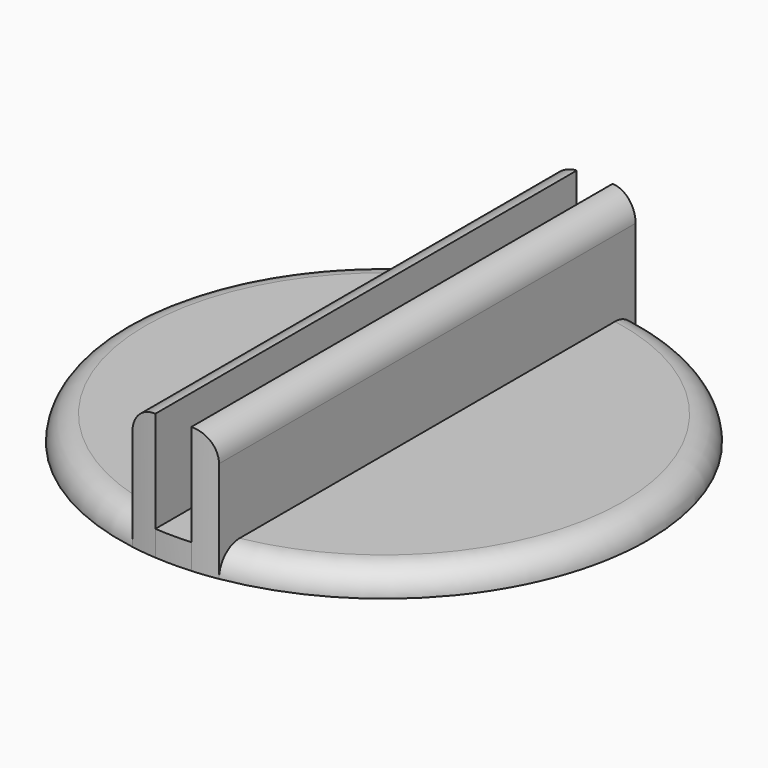
from build123d import *

# Parameters (mm, degrees)
F1_DEPTH      = 1.2
F2_DEPTH      = 6
F3_T2_ANGLE   = 188.6591090802
F3_2_T2_ANGLE = 188.6591090802
F3_3_T1_DEPTH = 30.6615084697
F3_4_T1_DEPTH = 30.6615084697


# Not quite as in the source:
# - a fillet or chamfer that OpenCascade refuses, or shapes differently, is made with other operations: its cross-section is extruded or revolved along the edge and cut away or added


with BuildPart() as f1:
    # F0 (on Top) → F1 (new body)
    with BuildSketch(Plane.XY):
        with BuildLine():
            Line((-2.05, -12.3307542348), (-2.05, 12.3307542348))
            ThreePointArc((-2.05, 12.3307542348), (-12.5, 0), (-2.05, -12.3307542348))
        make_face()
    extrude(amount=F1_DEPTH)

    # F3: fillet of radius 1.2 on 1 edges, made by hand

    # F3_s1 → F3_t2 (revolve, cut)
    with BuildSketch(Plane(origin=(0, 0, 0), x_dir=(0, 0, 1), z_dir=(0.997146325, -0.0754930889, 0))):
        with BuildLine():
            ThreePointArc((0, -12.5), (0.8485281374, -12.1485281374), (1.2, -11.3))
            Line((1.2, -11.3), (1.2, -12.5))
            Line((1.2, -12.5), (0, -12.5))
        make_face()
    revolve(axis=Axis((0, 0, 1.2), (0, 0, 1)), revolution_arc=F3_T2_ANGLE, mode=Mode.SUBTRACT)


with BuildPart() as f1b:
    # F0 (on Top) → F1, piece 2 (new body)
    with BuildSketch(Plane.XY):
        with BuildLine():
            Line((0.85, -12.4710665141), (0.85, 12.4710665141))
            ThreePointArc((0.85, 12.4710665141), (0, 12.5), (-0.85, 12.4710665141))
            Line((-0.85, 12.4710665141), (-0.85, -12.4710665141))
            ThreePointArc((-0.85, -12.4710665141), (0, -12.5), (0.85, -12.4710665141))
        make_face()
    extrude(amount=F1_DEPTH)


with BuildPart() as f1c:
    # F0 (on Top) → F1, piece 3 (new body)
    with BuildSketch(Plane.XY):
        with BuildLine():
            ThreePointArc((2.05, -12.3307542348), (9.5361155614, -8.0816149376), (12.5, 0))
            ThreePointArc((12.5, 0), (9.5361155614, 8.0816149376), (2.05, 12.3307542348))
            Line((2.05, 12.3307542348), (2.05, -12.3307542348))
        make_face()
    extrude(amount=F1_DEPTH)

    # F3#2: fillet of radius 1.2 on 1 edges, made by hand

    # F3_2_s1 → F3_2_t2 (revolve, cut)
    with BuildSketch(Plane(origin=(0, 0, 0), x_dir=(0, 0, 1), z_dir=(-0.997146325, -0.0754930889, 0))):
        with BuildLine():
            ThreePointArc((0, 12.5), (0.8485281374, 12.1485281374), (1.2, 11.3))
            Line((1.2, 11.3), (1.2, 12.5))
            Line((1.2, 12.5), (0, 12.5))
        make_face()
    revolve(axis=Axis((0, 0, 1.2), (0, 0, -1)), revolution_arc=F3_2_T2_ANGLE, mode=Mode.SUBTRACT)


with BuildPart() as f2:
    # F0 (on Top) → F2 (new body)
    with BuildSketch(Plane.XY):
        with BuildLine():
            Line((2.05, -12.3307542348), (2.05, 12.3307542348))
            ThreePointArc((2.05, 12.3307542348), (1.4516962092, 12.415416953), (0.85, 12.4710665141))
            Line((0.85, 12.4710665141), (0.85, -12.4710665141))
            ThreePointArc((0.85, -12.4710665141), (1.4516962092, -12.415416953), (2.05, -12.3307542348))
        make_face()
    extrude(amount=F2_DEPTH)

    # F3#3: fillet of radius 1.2 on 1 edges, made by hand

    # F3_3_s2 → F3_3_t1 (cut)
    with BuildSketch(Plane.XZ.offset(-15.3307542348)):
        with BuildLine():
            ThreePointArc((2.05, 4.8), (1.6985281374, 5.6485281374), (0.85, 6))
            Line((0.85, 6), (2.05, 6))
            Line((2.05, 6), (2.05, 4.8))
        make_face()
    extrude(amount=F3_3_T1_DEPTH, mode=Mode.SUBTRACT)


with BuildPart() as f2b:
    # F0 (on Top) → F2, piece 2 (new body)
    with BuildSketch(Plane.XY):
        with BuildLine():
            Line((-0.85, -12.4710665141), (-0.85, 12.4710665141))
            ThreePointArc((-0.85, 12.4710665141), (-1.4516962092, 12.415416953), (-2.05, 12.3307542348))
            Line((-2.05, 12.3307542348), (-2.05, -12.3307542348))
            ThreePointArc((-2.05, -12.3307542348), (-1.4516962092, -12.415416953), (-0.85, -12.4710665141))
        make_face()
    extrude(amount=F2_DEPTH)

    # F3#4: fillet of radius 1.2 on 1 edges, made by hand

    # F3_4_s2 → F3_4_t1 (cut)
    with BuildSketch(Plane.XZ.offset(-15.3307542348)):
        with BuildLine():
            ThreePointArc((-2.05, 4.8), (-1.6985281374, 5.6485281374), (-0.85, 6))
            Line((-0.85, 6), (-2.05, 6))
            Line((-2.05, 6), (-2.05, 4.8))
        make_face()
    extrude(amount=F3_4_T1_DEPTH, mode=Mode.SUBTRACT)


solid = Compound([f1.part, f1b.part, f1c.part, f2.part, f2b.part])
